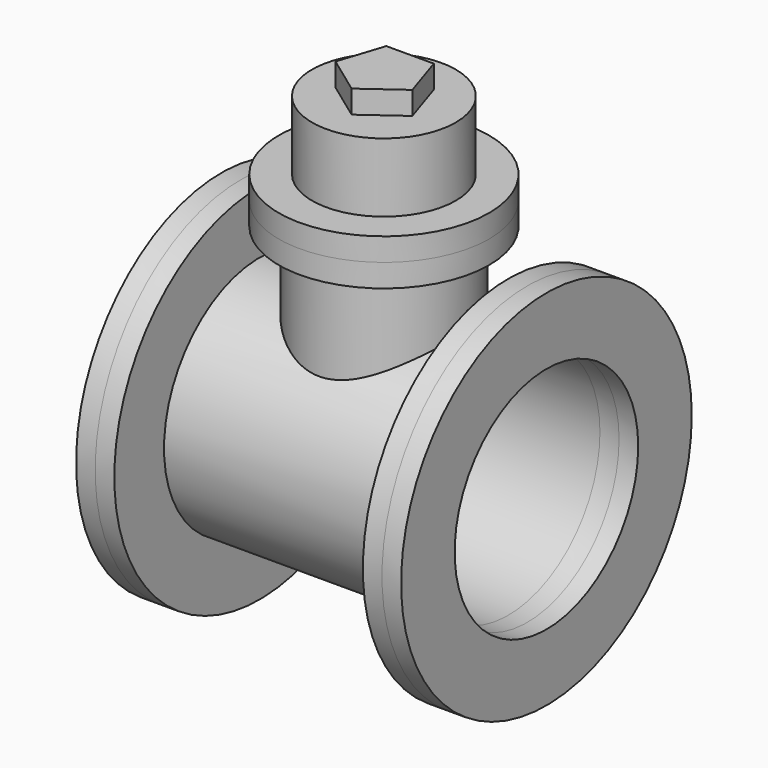
from build123d import *

# Parameters (mm, degrees)
F0_R      = 241.3
F0_R_2    = 152.4
F1_DEPTH  = 25.4
F3_R      = 241.3
F3_R_2    = 152.4
F4_DEPTH  = 25.4
F6_DEPTH  = 25.4
F7_DEPTH  = 25.4
F9_R      = 158.75
F9_R_2    = 152.4
F10_DEPTH = 330.2
F12_R     = 139.7
F13_DEPTH = 30.48
F14_R     = 107.3588969204
F15_REACH = 793.8778161324
F16_DEPTH = 30.48
F17_R     = 95.4249040927
F18_DEPTH = 91.44
F20_DEPTH = 30.48


with BuildPart() as f1:
    # F0 (on Right) → F1 (new body)
    with BuildSketch(Plane.YZ):
        Circle(F0_R)
        Circle(F0_R_2, mode=Mode.SUBTRACT)
    extrude(amount=F1_DEPTH)


with BuildPart() as f4:
    # F3 (on offset) → F4 (new body)
    with BuildSketch(Plane.YZ.offset(-330.2)):
        Circle(F3_R)
        Circle(F3_R_2, mode=Mode.SUBTRACT)
    extrude(amount=-F4_DEPTH)


with BuildPart() as f6:
    # F6 (new): a face of the model
    f6_faces = [f4.part.faces().sort_by_distance(p)[0] for p in [
        (-355.6, -234.475005348, 0),
    ]]
    extrude(f6_faces, amount=F6_DEPTH)


with BuildPart() as f7:
    # F7 (new): a face of the model
    f7_faces = [f1.part.faces().sort_by_distance(p)[0] for p in [
        (25.4, -234.475005348, 0),
    ]]
    extrude(f7_faces, amount=F7_DEPTH)


with BuildPart() as f1_1:
    add(f1.part)

    add(f4.part)  # F10 merges F4
    # F9 (on face) → F10 (join, through all)
    with BuildSketch(Plane.YZ.offset(-330.2)):
        Circle(F9_R)
        Circle(F9_R_2, mode=Mode.SUBTRACT)
    extrude(amount=F10_DEPTH)



with BuildPart() as f13:
    # F12 (on offset) → F13 (new body)
    with BuildSketch(Plane.XY.offset(279.4)):
        with Locations((-165.1, 0)):
            Circle(F12_R)
    extrude(amount=-F13_DEPTH)


with BuildPart() as f1_2:
    add(f1_1.part)

    add(f13.part)  # F15 merges F13
    f15_end = f1_2.faces().sort_by_distance((-165.1, -158.75, 0))[0]
    # F14 (on face) → F15 (join, up to a face of the model that its end follows)
    with BuildSketch(Plane(origin=(0, 0, 248.92), x_dir=(1, 0, 0), z_dir=(0, 0, -1))):
        with Locations((-165.1, 0)):
            Circle(F14_R)
    f15_long = extrude(amount=F15_REACH, mode=Mode.PRIVATE)
    add(split(f15_long, bisect_by=f15_end, keep=Keep.ALL, mode=Mode.PRIVATE).solids().sort_by_distance((-165.1, 0, 248.92))[0])


with BuildPart() as f16:
    # F16 (new): a face of the model
    f16_faces = [f1_2.part.faces().sort_by_distance(p)[0] for p in [
        (-165.1, 0, 279.4),
    ]]
    extrude(f16_faces, amount=F16_DEPTH)

    # F17 (on face) → F18 (join)
    with BuildSketch(Plane.XY.offset(309.88)):
        with Locations((-165.1, 0)):
            Circle(F17_R)
    extrude(amount=F18_DEPTH)

    # F19 (on face) → F20 (join)
    with BuildSketch(Plane.XY.offset(401.32)):
        Polygon((-133.5676910353, 43.4004999697), (-196.6323089647, 43.4004999697), (-216.1203476486, -16.5775158597), (-165.1, -53.6459682201), (-114.0796523514, -16.5775158597), align=None)
    extrude(amount=F20_DEPTH)


solid = Compound([f6.part, f7.part, f1_2.part, f16.part])
